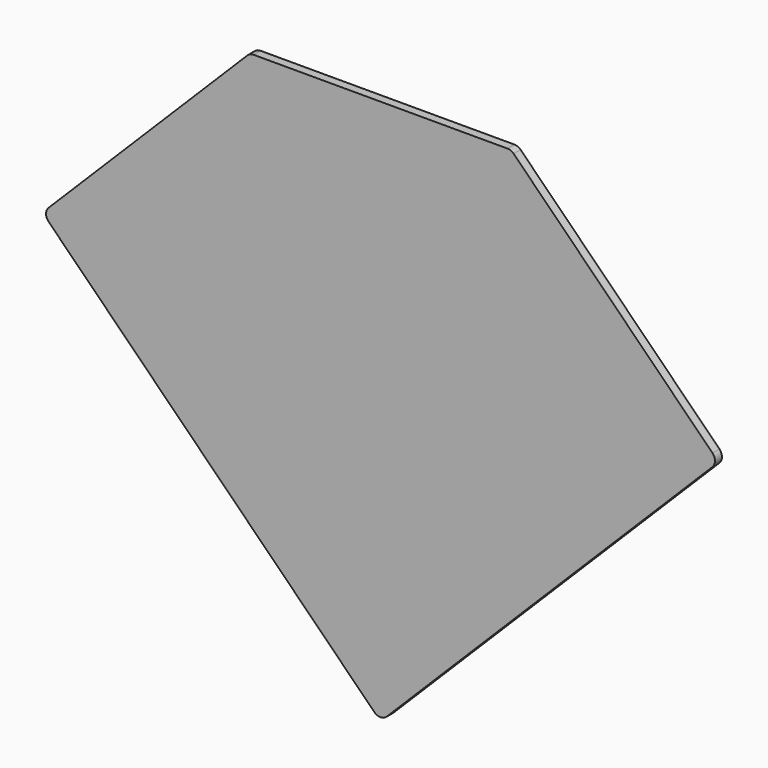
from build123d import *

# Parameters (mm, degrees)
F1_DEPTH = 10


# Not quite as in the source:
# - a feature names something its author has since deleted; it is built from what else it names


with BuildPart() as f1:
    # F0 (on Front) → F1 (new body)
    with BuildSketch(Plane.XZ):
        with BuildLine():
            Line((-152.9289321881, 147.0710678119), (-300, 0))
            Line((-300, 0), (-381.3172798365, -81.3172798365))
            ThreePointArc((-381.3172798365, -81.3172798365), (-384.2462120246, -88.3883476483), (-381.3172798365, -95.4594154602))
            Line((-381.3172798365, -95.4594154602), (-155.0431098568, -321.7335854399))
            Line((-155.0431098568, -321.7335854399), (-7.0710678119, -469.7056274848))
            ThreePointArc((-7.0710678119, -469.7056274848), (0, -472.6345596729), (7.0710678119, -469.7056274848))
            Line((7.0710678119, -469.7056274848), (155.0431098568, -321.7335854399))
            Line((155.0431098568, -321.7335854399), (381.3172798365, -95.4594154602))
            ThreePointArc((381.3172798365, -95.4594154602), (384.2462120246, -88.3883476483), (381.3172798365, -81.3172798365))
            Line((381.3172798365, -81.3172798365), (300, 0))
            Line((300, 0), (152.9289321881, 147.0710678119))
            ThreePointArc((152.9289321881, 147.0710678119), (149.6846986999, 149.2387953251), (145.8578643763, 150))
            Line((145.8578643763, 150), (-145.8578643763, 150))
            ThreePointArc((-145.8578643763, 150), (-149.6846986999, 149.2387953251), (-152.9289321881, 147.0710678119))
        make_face()
    extrude(amount=F1_DEPTH)


solid = f1.part
